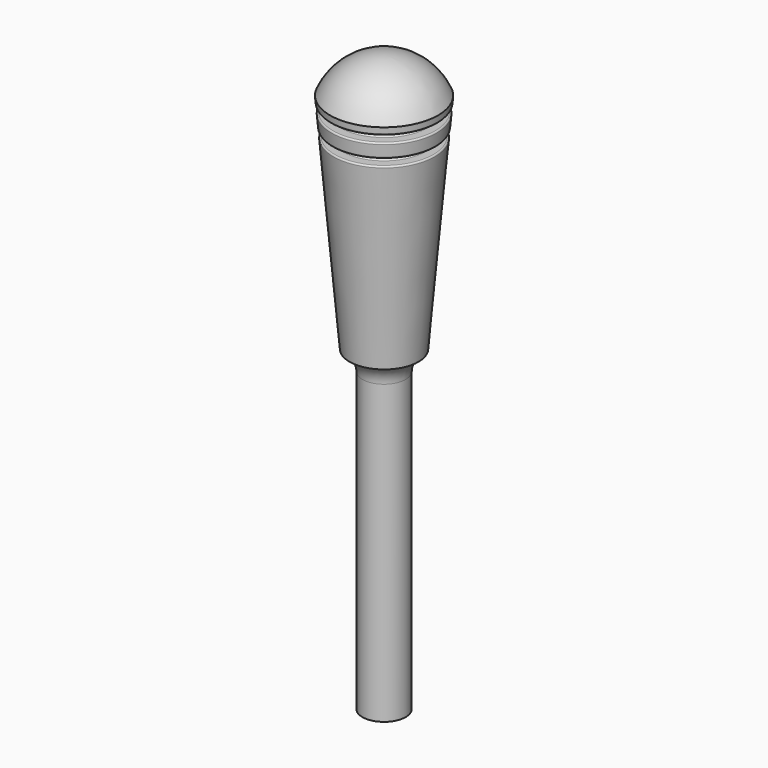
from build123d import *

# Parameters (mm, degrees)
F3_R = 0.1


# Not quite as in the source:
# - a fillet or chamfer that OpenCascade refuses, or shapes differently, is made with other operations: its cross-section is extruded or revolved along the edge and cut away or added


with BuildPart() as f1:
    # F0 (on Front) → F1 (revolve)
    with BuildSketch(Plane.XZ):
        with BuildLine():
            Line((0, 21.6683513987), (0, 0))
            Line((0, 0), (1.5, 0))
            Line((1.5, 0), (1.5, 22))
            Line((1.5, 22), (2.3939257153, 22))
            Line((2.3939257153, 22), (3.5314448016, 35.001902651))
            Line((3.5314448016, 35.001902651), (2.7814448016, 35.001902651))
            Line((2.7814448016, 35.001902651), (2.8250226729, 35.5))
            Line((2.8250226729, 35.5), (3.5750226729, 35.5))
            Line((3.5750226729, 35.5), (3.6621784157, 36.4961946981))
            Line((3.6621784157, 36.4961946981), (2.9121784157, 36.4961946981))
            Line((2.9121784157, 36.4961946981), (2.9557562871, 36.9942920471))
            Line((2.9557562871, 36.9942920471), (3.7057562871, 36.9942920471))
            Line((3.7057562871, 36.9942920471), (3.75, 37.5))
            ThreePointArc((3.75, 37.5), (2.2534695472, 39.3177043207), (0, 40))
            Line((0, 40), (0, 37.5))
            Line((0, 37.5), (0, 21.6683513987))
        make_face()
    revolve(axis=Axis((0, 0, 29.5841756993), (0, 0, 1)))

    # F2: fillet of radius 1.5 on 1 edges, made by hand

    # F2_s1 → F2_t2 (revolve)
    with BuildSketch(Plane.XZ):
        with BuildLine():
            ThreePointArc((1.5, 20.627894333), (1.7431962311, 21.4467009564), (2.3939257153, 22))
            Line((2.3939257153, 22), (2.3818042297, 22.0274421133))
            ThreePointArc((2.3818042297, 22.0274421133), (1.9469628577, 22.03), (1.5, 22.03))
            Line((1.5, 22.03), (1.47, 22))
            Line((1.47, 22), (1.47, 20.627894333))
            Line((1.47, 20.627894333), (1.5, 20.627894333))
        make_face()
    revolve(axis=Axis((0, 0, 22), (0, 0, 1)))

    # F3
    f3_edges = [f1.edges().sort_by_distance(p)[0] for p in [
        (-2.825023, 0, 35.5),
        (-2.781445, 0, 35.001903),
        (-3.531445, 0, 35.001903),
        (-3.575023, 0, 35.5),
        (-2.912178, 0, 36.496195),
        (-2.955756, 0, 36.994292),
        (2.933967, 0, 36.745243),
        (-3.662178, 0, 36.496195),
        (-3.705756, 0, 36.994292),
    ]]
    fillet(f3_edges, radius=F3_R)


solid = f1.part
